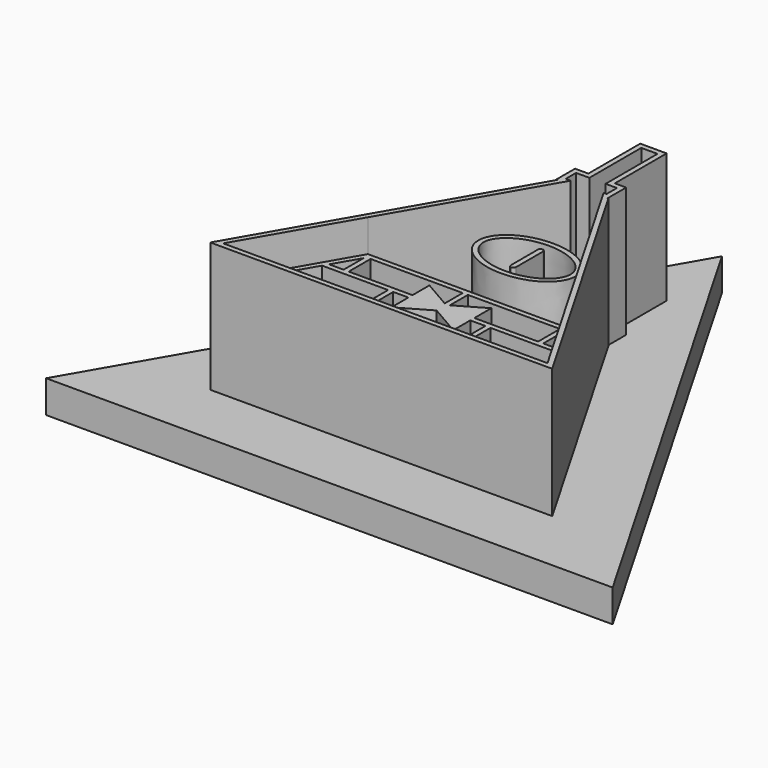
from build123d import *

# Parameters (mm, degrees)
F0_W     = 18.05
F0_H     = 5.358
F1_DEPTH = 19.05
F2_DEPTH = 25.4
F4_DEPTH = 6.35


# Not quite as in the source:
# - the dataset's text gives a spline's control points without its knots; the knots are read off the source's solid


with BuildPart() as f1:
    # F0 (on Top) → F1 (new body)
    with BuildSketch(Plane.XY):
        Polygon((-73.402151112, 4.5771139196), (-78.1832148198, 4.5771139196), (-82.1426829659, -2.2808860804), (-73.402151112, -2.2808860804), (-63.877151112, -2.2808860804), (-63.877151112, 4.5771139196), align=None)
        Polygon((-64.377151112, -1.7808860804), (-80.6993072929, -1.7808860804), (-77.317189416, 4.0771139196), (-64.377151112, 4.0771139196), align=None, mode=Mode.SUBTRACT)
        Polygon((-73.402151112, -2.2808860804), (-82.1426829659, -2.2808860804), (-86.102151112, -9.1388860804), (-73.402151112, -9.1388860804), align=None)
        Polygon((-84.3701003044, -8.1388860804), (-81.2766575621, -2.7808860804), (-73.902151112, -2.7808860804), (-73.902151112, -8.1388860804), align=None, mode=Mode.SUBTRACT)
        Polygon((-63.877151112, -2.2808860804), (-73.402151112, -2.2808860804), (-73.402151112, -9.1388860804), (-54.352151112, -9.1388860804), (-54.352151112, -2.2808860804), align=None)
        with Locations((-63.877151112, -5.4598860804)):
            Rectangle(F0_W, F0_H, mode=Mode.SUBTRACT)
        Polygon((-35.302151112, 11.4351139196), (-73.402151112, 11.4351139196), (-73.402151112, 4.5771139196), (-63.877151112, 4.5771139196), (-63.877151112, -2.2808860804), (-54.352151112, -2.2808860804), (-44.827151112, -2.2808860804), (-44.827151112, 4.5771139196), (-35.302151112, 4.5771139196), align=None)
        Polygon((-48.2928307031, -0.0759368879), (-48.2928307031, 4.0771139196), (-45.327151112, 4.0771139196), (-45.327151112, -1.7808860804), (-63.377151112, -1.7808860804), (-63.377151112, 4.0771139196), (-60.4114715209, 4.0771139196), (-60.4114715209, -0.0759368879), (-54.352151112, 3.4224133812), align=None, mode=Mode.SUBTRACT)
        Polygon((-60.4114715209, 9.2301647272), (-60.4114715209, 5.0771139196), (-72.902151112, 5.0771139196), (-72.902151112, 10.4351139196), (-54.852151112, 10.4351139196), (-54.852151112, 6.0204895926), align=None, mode=Mode.SUBTRACT)
        Polygon((-35.802151112, 5.0771139196), (-48.2928307031, 5.0771139196), (-48.2928307031, 9.2301647272), (-53.852151112, 6.0204895926), (-53.852151112, 10.4351139196), (-35.802151112, 10.4351139196), align=None, mode=Mode.SUBTRACT)
        Polygon((-73.402151112, 11.4351139196), (-74.2237466737, 11.4351139196), (-78.1832148198, 4.5771139196), (-73.402151112, 4.5771139196), align=None)
        Polygon((-73.902151112, 5.0771139196), (-76.7398391468, 5.0771139196), (-73.902151112, 9.992133772), align=None, mode=Mode.SUBTRACT)
        Polygon((-34.4805555503, 11.4351139196), (-35.302151112, 11.4351139196), (-35.302151112, 4.5771139196), (-30.5210874042, 4.5771139196), align=None)
        Polygon((-34.802151112, 10.1431388709), (-31.8772802426, 5.0771139196), (-34.802151112, 5.0771139196), align=None, mode=Mode.SUBTRACT)
        Polygon((-30.5210874042, 4.5771139196), (-35.302151112, 4.5771139196), (-44.827151112, 4.5771139196), (-44.827151112, -2.2808860804), (-35.302151112, -2.2808860804), (-26.5616192581, -2.2808860804), align=None)
        Polygon((-31.387112808, 4.0771139196), (-28.0049949311, -1.7808860804), (-44.327151112, -1.7808860804), (-44.327151112, 4.0771139196), align=None, mode=Mode.SUBTRACT)
        Polygon((-22.602151112, -9.1388860804), (-26.5616192581, -2.2808860804), (-35.302151112, -2.2808860804), (-35.302151112, -9.1388860804), align=None)
        Polygon((-34.802151112, -2.7808860804), (-27.4276446619, -2.7808860804), (-24.3342019195, -8.1388860804), (-34.802151112, -8.1388860804), align=None, mode=Mode.SUBTRACT)
        Polygon((-54.352151112, -2.2808860804), (-54.352151112, -9.1388860804), (-35.302151112, -9.1388860804), (-35.302151112, -2.2808860804), (-44.827151112, -2.2808860804), align=None)
        with Locations((-44.827151112, -5.4598860804)):
            Rectangle(F0_W, F0_H, mode=Mode.SUBTRACT)
    extrude(amount=F1_DEPTH)

    # F0 (on Top) → F2 (join)
    with BuildSketch(Plane.XY):
        Polygon((-56.939651112, 43.7939179328), (-59.5488287793, 43.7939179328), (-59.5488287793, 39.2539179328), (-59.3172532265, 39.2539179328), (-87.8342019195, -10.1388860804), (-20.8701003044, -10.1388860804), (-49.3870489975, 39.2539179328), (-49.542151112, 39.2539179328), (-49.542151112, 43.7939179328), (-51.764651112, 43.7939179328), (-51.764651112, 56.4939179328), (-56.939651112, 56.4939179328), align=None)
        Polygon((-74.2237466737, 11.4351139196), (-57.5852024189, 40.2539179328), (-58.5488287793, 40.2539179328), (-58.5488287793, 42.7939179328), (-55.939651112, 42.7939179328), (-55.939651112, 55.4939179328), (-52.764651112, 55.4939179328), (-52.764651112, 42.7939179328), (-50.542151112, 42.7939179328), (-50.542151112, 40.2539179328), (-51.119099805, 40.2539179328), (-34.4805555503, 11.4351139196), (-30.5210874042, 4.5771139196), (-26.5616192581, -2.2808860804), (-22.602151112, -9.1388860804), (-35.302151112, -9.1388860804), (-54.352151112, -9.1388860804), (-73.402151112, -9.1388860804), (-86.102151112, -9.1388860804), (-82.1426829659, -2.2808860804), (-78.1832148198, 4.5771139196), align=None, mode=Mode.SUBTRACT)
    extrude(amount=F2_DEPTH)


with BuildPart() as f1b:
    # F0 (on Top) → F1, piece 2 (new body)
    with BuildSketch(Plane.XY):
        with BuildLine():
            add(Edge.make_bspline(
                [(-54.352145642, 19.1837270599), (-37.8543616999, 19.1837270599), (-46.103253671, 28.7087270599), (-54.352145642, 38.2337270599), (-62.6010376131, 28.7087270599), (-70.8499295841, 19.1837270599), (-54.352145642, 19.1837270599)],
                knots=[4.7123889804, 4.7123889804, 4.7123889804, 6.8067840828, 6.8067840828, 8.9011791852, 8.9011791852, 10.9955742876, 10.9955742876, 10.9955742876], degree=2, weights=[1, 0.5, 1, 0.5, 1, 0.5, 1]))
        make_face()
        with BuildLine():
            add(Edge.make_bspline(
                [(-45.827145642, 25.5337270599), (-45.827145642, 25.8519377152), (-45.9208714076, 26.4883590256), (-46.3482817791, 27.4376066909), (-47.0906705746, 28.3694216685), (-48.1278583866, 29.2134440557), (-49.4278608435, 29.9276027455), (-50.9536840842, 30.4720106822), (-52.334286038, 30.7509003907), (-53.4791973585, 30.8645462988), (-54.352145642, 30.8933174405), (-55.2250939256, 30.8645462988), (-56.3700052461, 30.7509003907), (-57.7506071999, 30.4720106822), (-59.2764304406, 29.9276027455), (-60.5764328975, 29.2134440557), (-61.6136207095, 28.3694216685), (-62.3560095049, 27.4376066909), (-62.7834198764, 26.4883590256), (-62.9240085248, 25.5337270599), (-62.7834198764, 24.5790950943), (-62.3560095049, 23.6298474289), (-61.6136207095, 22.6980324514), (-60.5764328975, 21.8540100641), (-59.2764304406, 21.1398513743), (-57.7506071999, 20.5954434377), (-56.3700052461, 20.3165537291), (-55.2250939256, 20.2029078211), (-54.352145642, 20.1741366794), (-53.4791973585, 20.2029078211), (-52.334286038, 20.3165537291), (-50.9536840842, 20.5954434377), (-49.4278608435, 21.1398513743), (-48.1278583866, 21.8540100641), (-47.0906705746, 22.6980324514), (-46.3482817791, 23.6298474289), (-45.9208714076, 24.5790950943), (-45.827145642, 25.2155164047), (-45.827145642, 25.5337270599)],
                knots=[0, 0, 0, 0, 0.03125, 0.0625, 0.09375, 0.125, 0.15625, 0.1875, 0.21875, 0.234375, 0.25, 0.265625, 0.28125, 0.3125, 0.34375, 0.375, 0.40625, 0.4375, 0.46875, 0.5, 0.53125, 0.5625, 0.59375, 0.625, 0.65625, 0.6875, 0.71875, 0.734375, 0.75, 0.765625, 0.78125, 0.8125, 0.84375, 0.875, 0.90625, 0.9375, 0.96875, 1, 1, 1, 1], degree=3))
        make_face(mode=Mode.SUBTRACT)
    extrude(amount=F1_DEPTH)


with BuildPart() as f1c:
    # F0 (on Top) → F1, piece 3 (new body)
    with BuildSketch(Plane.XY):
        with BuildLine():
            ThreePointArc((-54.352145642, 29.3437270599), (-54.7113558869, 29.1949373048), (-54.860145642, 28.8357270599))
            Line((-54.860145642, 28.8357270599), (-54.860145642, 22.2317270599))
            ThreePointArc((-54.860145642, 22.2317270599), (-54.7113558869, 21.8725168151), (-54.352145642, 21.7237270599))
            ThreePointArc((-54.352145642, 21.7237270599), (-53.9929353972, 21.8725168151), (-53.844145642, 22.2317270599))
            Line((-53.844145642, 22.2317270599), (-53.844145642, 28.8357270599))
            ThreePointArc((-53.844145642, 28.8357270599), (-53.9929353972, 29.1949373048), (-54.352145642, 29.3437270599))
        make_face()
    extrude(amount=F1_DEPTH)


with BuildPart() as f4:
    # F3 (on face) → F4 (new body)
    with BuildSketch(Plane.XY):
        Polygon((-109.8312471757, -22.8388860804), (1.1269449517, -22.8388860804), (-54.352151112, 73.2537270599), align=None)
        Polygon((-59.5488287793, 43.7939179328), (-56.939651112, 43.7939179328), (-56.939651112, 56.4939179328), (-51.764651112, 56.4939179328), (-51.764651112, 43.7939179328), (-49.542151112, 43.7939179328), (-49.542151112, 39.2539179328), (-49.3870489975, 39.2539179328), (-20.8701003044, -10.1388860804), (-87.8342019195, -10.1388860804), (-59.3172532265, 39.2539179328), (-59.5488287793, 39.2539179328), align=None, mode=Mode.SUBTRACT)
        Polygon((-56.939651112, 56.4939179328), (-56.939651112, 43.7939179328), (-59.5488287793, 43.7939179328), (-59.5488287793, 39.2539179328), (-59.3172532265, 39.2539179328), (-87.8342019195, -10.1388860804), (-20.8701003044, -10.1388860804), (-49.3870489975, 39.2539179328), (-49.542151112, 39.2539179328), (-49.542151112, 43.7939179328), (-51.764651112, 43.7939179328), (-51.764651112, 56.4939179328), align=None)
        Polygon((-78.1832148198, 4.5771139196), (-74.2237466737, 11.4351139196), (-57.5852024189, 40.2539179328), (-58.5488287793, 40.2539179328), (-58.5488287793, 42.7939179328), (-55.939651112, 42.7939179328), (-55.939651112, 55.4939179328), (-52.764651112, 55.4939179328), (-52.764651112, 42.7939179328), (-50.542151112, 42.7939179328), (-50.542151112, 40.2539179328), (-51.119099805, 40.2539179328), (-34.4805555503, 11.4351139196), (-30.5210874042, 4.5771139196), (-26.5616192581, -2.2808860804), (-22.602151112, -9.1388860804), (-35.302151112, -9.1388860804), (-54.352151112, -9.1388860804), (-73.402151112, -9.1388860804), (-86.102151112, -9.1388860804), (-82.1426829659, -2.2808860804), align=None, mode=Mode.SUBTRACT)
        Polygon((-57.5852024189, 40.2539179328), (-74.2237466737, 11.4351139196), (-78.1832148198, 4.5771139196), (-82.1426829659, -2.2808860804), (-86.102151112, -9.1388860804), (-73.402151112, -9.1388860804), (-54.352151112, -9.1388860804), (-35.302151112, -9.1388860804), (-22.602151112, -9.1388860804), (-26.5616192581, -2.2808860804), (-30.5210874042, 4.5771139196), (-34.4805555503, 11.4351139196), (-51.119099805, 40.2539179328), (-50.542151112, 40.2539179328), (-50.542151112, 42.7939179328), (-52.764651112, 42.7939179328), (-52.764651112, 55.4939179328), (-55.939651112, 55.4939179328), (-55.939651112, 42.7939179328), (-58.5488287793, 42.7939179328), (-58.5488287793, 40.2539179328), align=None)
        with BuildLine():
            ThreePointArc((-63.6885240674, 21.3321540505), (-53.5401728786, 17.0166304748), (-43.5974113792, 21.7867740102))
            Line((-43.5974113792, 21.7867740102), (-38.8624295592, 13.6320823804))
            Line((-38.8624295592, 13.6320823804), (-69.1316798329, 13.6320823804))
            Line((-69.1316798329, 13.6320823804), (-63.6885240674, 21.3321540505))
        make_face(mode=Mode.SUBTRACT)
    extrude(amount=-F4_DEPTH)


solid = Compound([f1.part, f1b.part, f1c.part, f4.part])
